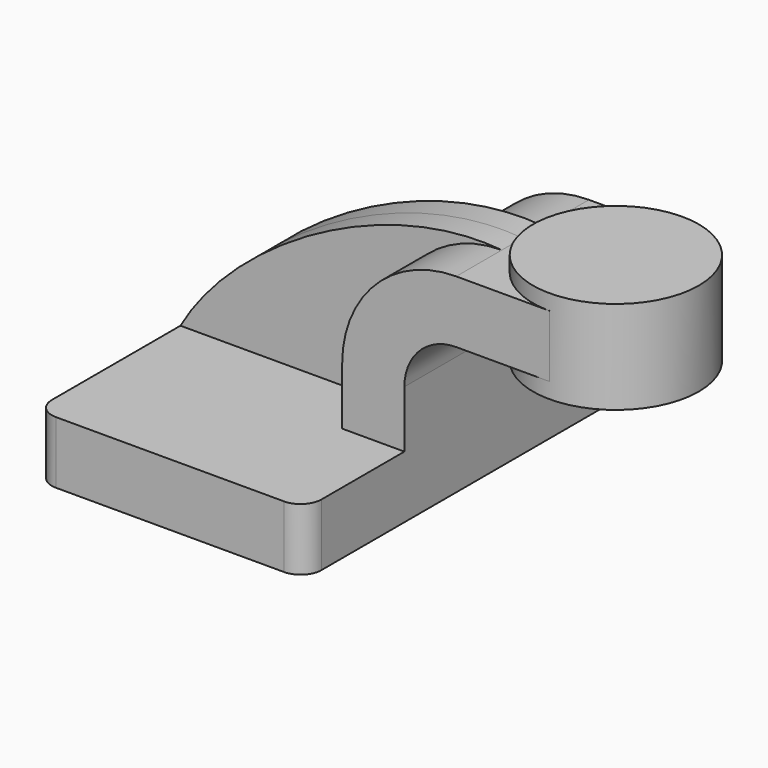
from build123d import *

# Parameters (mm, degrees)
F1_DEPTH = 63.5
F0_W     = 25.4
F0_H     = 19.05
F2_DEPTH = 25.4
F3_DEPTH = 7.9375
F5_R     = 6.35


with BuildPart() as f1:
    # F0 (on Front) → F1 (new body, symmetric)
    with BuildSketch(Plane.XZ):
        Polygon((-49.2188632803, -9.525), (33.3311367197, -9.525), (33.3311367197, 9.525), (14.2811367197, 9.525), (-49.2188632803, 9.525), align=None)
    extrude(amount=F1_DEPTH, both=True)

    # F0 (on Front) → F2 (join, symmetric)
    with BuildSketch(Plane.XZ):
        with BuildLine():
            Line((14.2811367197, 9.525), (33.3311367197, 9.525))
            Line((33.3311367197, 9.525), (33.3311367197, 27.0002))
            ThreePointArc((33.3311367197, 27.0002), (37.9808165684, 38.2255201513), (49.2061367197, 42.8752))
            Line((49.2061367197, 42.8752), (52.3811367197, 42.8752))
            Line((52.3811367197, 42.8752), (52.3811367197, 61.9252))
            Line((52.3811367197, 61.9252), (49.2061367197, 61.9252))
            ThreePointArc((49.2061367197, 61.9252), (24.5104323868, 51.6959043329), (14.2811367197, 27.0002))
            Line((14.2811367197, 27.0002), (14.2811367197, 9.525))
        make_face()
        with Locations((65.0811367197, 52.4002)):
            Rectangle(F0_W, F0_H)
    extrude(amount=F2_DEPTH, both=True)

    # F0 (on Front) → F3 (join, symmetric)
    with BuildSketch(Plane.XZ):
        with BuildLine():
            add(Edge.make_bspline(
                [(-49.2188632803, 9.525), (-32.7156037092, 38.7257821858), (12.8561593592, 65.2922838926), (49.2061367197, 61.9252)],
                knots=[0, 0, 0, 0, 111.5045361635, 111.5045361635, 111.5045361635, 111.5045361635], degree=3))
            Line((-49.2188632803, 9.525), (14.2811367197, 9.525))
            Line((14.2811367197, 9.525), (14.2811367197, 27.0002))
            ThreePointArc((14.2811367197, 27.0002), (24.5104323868, 51.6959043329), (49.2061367197, 61.9252))
        make_face()
    extrude(amount=F3_DEPTH, both=True)

    # F5
    f5_edges = [f1.edges().sort_by_distance(p)[0] for p in [
        (-49.218863, -63.5, 0),
        (33.331137, -63.5, 0),
        (33.331137, 63.5, 0),
        (-49.218863, 63.5, 0),
    ]]
    fillet(f5_edges, radius=F5_R)


with BuildPart() as f4:
    # F0 (on Front) → F4 (revolve)
    with BuildSketch(Plane.XZ):
        Polygon((77.7811367197, 66.675), (77.7811367197, 61.9252), (77.7811367197, 42.8752), (77.7811367197, 38.1), (103.1811367197, 38.1), (103.1811367197, 66.675), align=None)
    revolve(axis=Axis((77.7811367197, 0, 52.3875), (0, 0, 1)))


solid = Compound([f1.part, f4.part])
